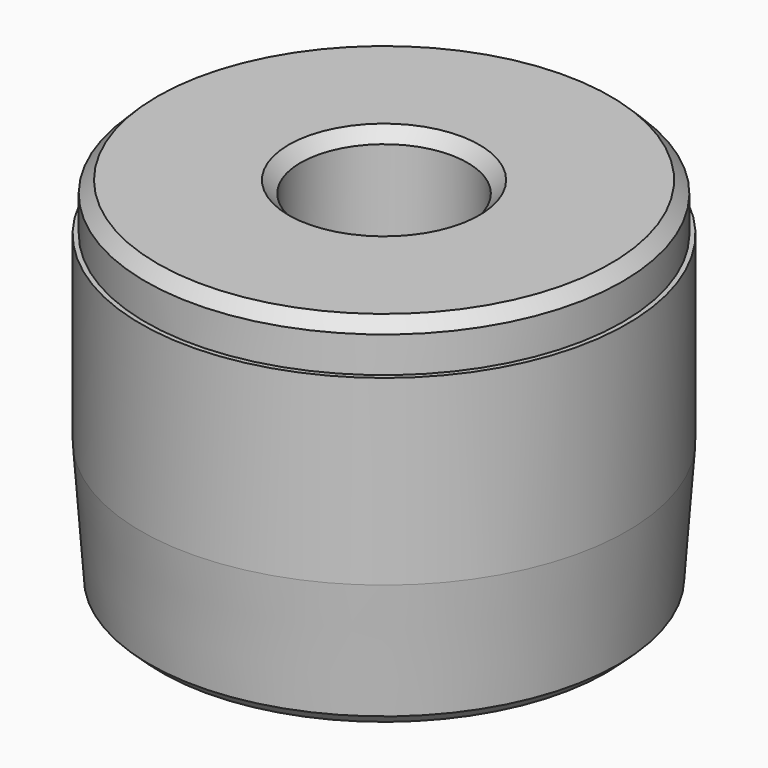
from build123d import *


# Not quite as in the source:
# - a fillet or chamfer that OpenCascade refuses, or shapes differently, is made with other operations: its cross-section is extruded or revolved along the edge and cut away or added


with BuildPart() as f1:
    # F0 (on Front) → F1 (revolve)
    with BuildSketch(Plane.XZ):
        Polygon((-3.5, -0.575), (-3.5, 7.575), (-10, 7.575), (-10, 5.575), (-10.2, 5.575), (-10.2, -2.075), (-9.8, -7.575), (-5.5, -7.575), (-5.5, -0.575), align=None)
    revolve(axis=Axis((0, 0, 0.3696661443), (0, 0, -1)))

    # F2: chamfer of 0.5 on 4 edges, made by hand

    # F2_s1 → F2_t2 (revolve, cut)
    with BuildSketch(Plane.XZ):
        Polygon((-6, -7.575), (-5.5, -7.075), (-5.5, -7.575), align=None)
    revolve(axis=Axis((0, 0, -7.575), (0, 0, -1)), mode=Mode.SUBTRACT)

    # F2_s3 → F2_t4 (revolve, cut)
    with BuildSketch(Plane.XZ):
        Polygon((-9.8337259747, -7.1112678479), (-9.3350430662, -7.575), (-9.8, -7.575), align=None)
    revolve(axis=Axis((0, 0, -7.575), (0, 0, -1)), mode=Mode.SUBTRACT)

    # F2_s5 → F2_t6 (revolve, cut)
    with BuildSketch(Plane.XZ):
        Polygon((-9.5, 7.575), (-10, 7.075), (-10, 7.575), align=None)
    revolve(axis=Axis((0, 0, 7.575), (0, 0, -1)), mode=Mode.SUBTRACT)

    # F2_s7 → F2_t8 (revolve, cut)
    with BuildSketch(Plane.XZ):
        Polygon((-3.5, 7.075), (-4, 7.575), (-3.5, 7.575), align=None)
    revolve(axis=Axis((0, 0, 7.575), (0, 0, -1)), mode=Mode.SUBTRACT)


solid = f1.part
